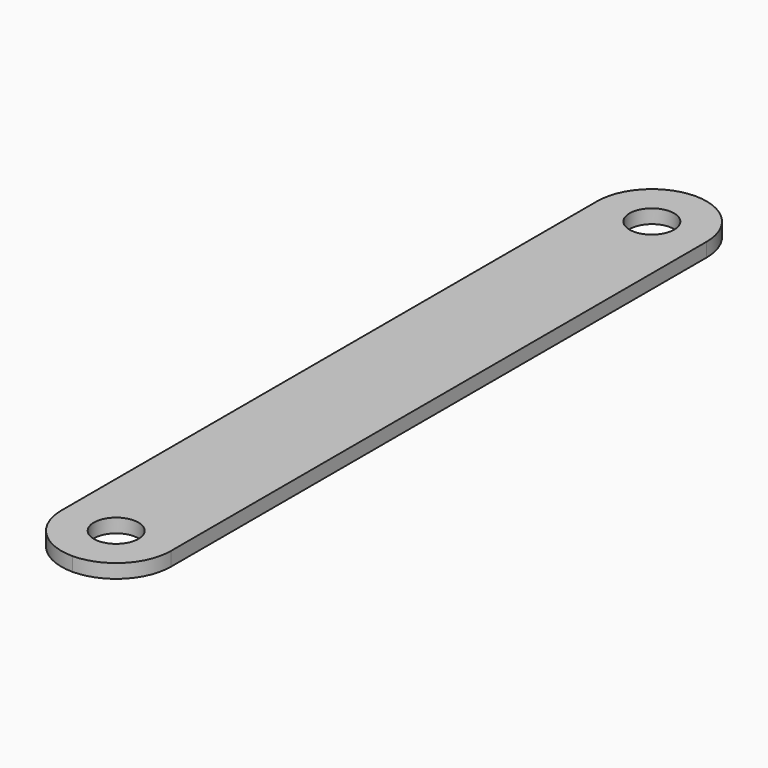
from build123d import *

# Parameters (mm, degrees)
F0_R     = 5.08
F1_DEPTH = 3.175


# Not quite as in the source:
# - a length typed as a fraction of an inch, garbled in the dataset ("3 / 203.2 mm" for 3/8 in), is restored


with BuildPart() as f1:
    # F0 (on Top) → F1 (new body)
    with BuildSketch(Plane.XY):
        with BuildLine():
            Line((12.5, -76.4), (12.5, 76.4))
            ThreePointArc((12.5, 76.4), (8.8388347648, 85.2388347648), (0, 88.9))
            ThreePointArc((0, 88.9), (-8.8388347648, 85.2388347648), (-12.5, 76.4))
            Line((-12.5, 76.4), (-12.5, -76.4))
            ThreePointArc((-12.5, -76.4), (-8.8388347648, -85.2388347648), (0, -88.9))
            ThreePointArc((0, -88.9), (8.8388347648, -85.2388347648), (12.5, -76.4))
        make_face()
        with Locations((0, -76.4)):
            Circle(F0_R, mode=Mode.SUBTRACT)
        with Locations((0, 76.4)):
            Circle(F0_R, mode=Mode.SUBTRACT)
    extrude(amount=F1_DEPTH)


solid = f1.part
